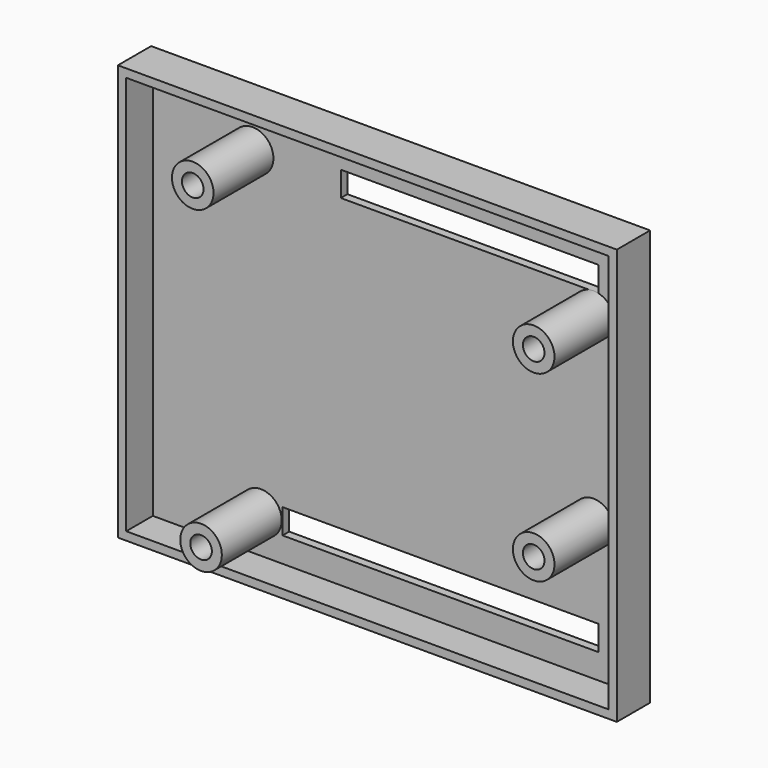
from build123d import *

# Parameters (mm, degrees)
F0_W     = 76.2
F0_H     = 63.5
F1_DEPTH = 6.35
F2_T     = -1.27
F3_R     = 3.175
F3_R_2   = 1.651
F4_DEPTH = 11.43
F5_W     = 48.26
F5_H     = 3.81
F5_W_2   = 39.37
F6_DEPTH = 1.27


# Not quite as in the source:
# - a feature names something its author has since deleted; it is built from what else it names


with BuildPart() as f1:
    # F0 (on Front) → F1 (new body)
    with BuildSketch(Plane.XZ):
        with Locations((38.1, 31.75)):
            Rectangle(F0_W, F0_H)
    extrude(amount=F1_DEPTH)

    # F2
    f2_openings = [f1.faces().sort_by_distance(p)[0] for p in [
        (38.1, -6.35, 31.75),
    ]]
    offset(amount=F2_T, openings=f2_openings)

    # F3 (on face) → F4 (join)
    with BuildSketch(Plane.XZ.offset(1.27)):
        with Locations((16.51, 55.3212)):
            Circle(F3_R)
        with Locations((16.51, 55.3212)):
            Circle(F3_R_2, mode=Mode.SUBTRACT)
        with Locations((68.58, 50.2412)):
            Circle(F3_R)
        with Locations((68.58, 50.2412)):
            Circle(F3_R_2, mode=Mode.SUBTRACT)
        with Locations((68.58, 22.3012)):
            Circle(F3_R)
        with Locations((68.58, 22.3012)):
            Circle(F3_R_2, mode=Mode.SUBTRACT)
        with Locations((17.78, 7.0612)):
            Circle(F3_R)
        with Locations((17.78, 7.0612)):
            Circle(F3_R_2, mode=Mode.SUBTRACT)
    extrude(amount=F4_DEPTH)

    # F5 (on face) → F6 (cut)
    with BuildSketch(Plane(origin=(0, 0, 0), x_dir=(-1, 0, 0), z_dir=(0, 1, 0))):
        with Locations((-45.212, 6.985)):
            Rectangle(F5_W, F5_H)
        with Locations((-49.657, 55.245)):
            Rectangle(F5_W_2, F5_H)
    extrude(amount=-F6_DEPTH, mode=Mode.SUBTRACT)


solid = f1.part
